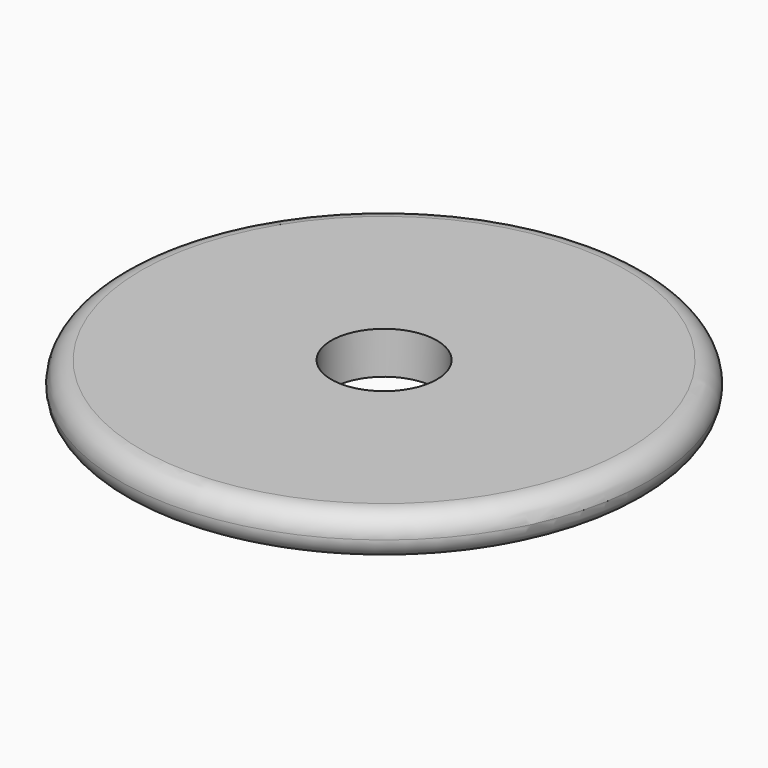
from build123d import *

# Parameters (mm, degrees)
F0_R     = 12.5
F0_R_2   = 2.5
F1_DEPTH = 2
F2_R     = 1
F3_R     = 0.99999


# Not quite as in the source:
# - a fillet or chamfer is up to 0.001 mm smaller than in the source, because OpenCascade refuses the exact size


with BuildPart() as f1:
    # F0 (on Top) → F1 (new body)
    with BuildSketch(Plane.XY):
        Circle(F0_R)
        Circle(F0_R_2, mode=Mode.SUBTRACT)
    extrude(amount=F1_DEPTH)

    # F2
    f2_edges = [f1.edges().sort_by_distance(p)[0] for p in [
        (-12.5, 0, 2),
    ]]
    fillet(f2_edges, radius=F2_R)

    # F3 (radius 1 in the source; OpenCascade refuses exactly that, so slightly less here)
    f3_edges = [f1.edges().sort_by_distance(p)[0] for p in [
        (-12.5, 0, 0),
    ]]
    fillet(f3_edges, radius=F3_R)


solid = f1.part
